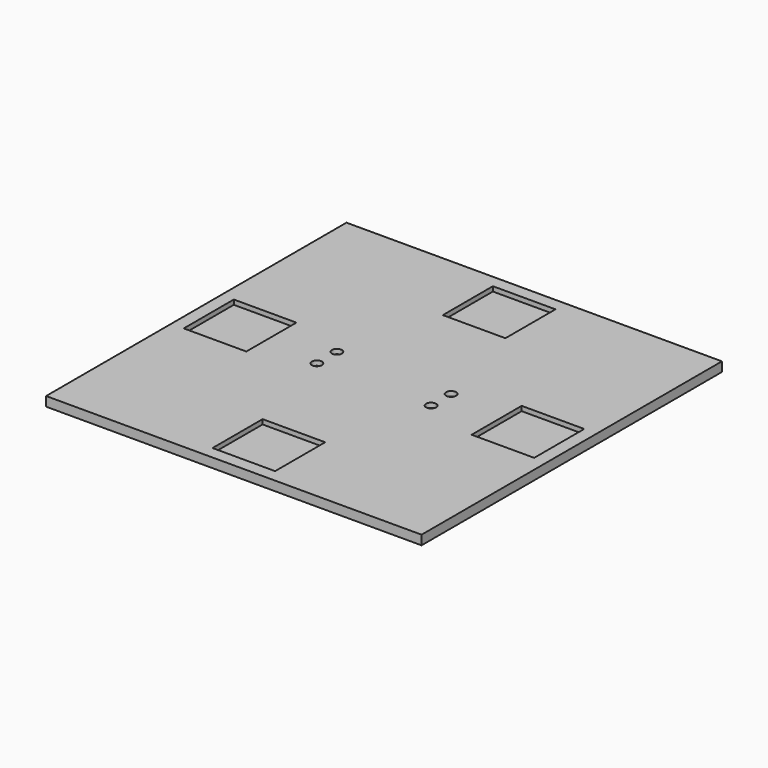
from build123d import *

# Parameters (mm, degrees)
F0_W             = 120
F0_H             = 120
F1_DEPTH         = 1.5
F5_W             = 120
F5_H             = 120
F5_W_2           = 112
F5_H_2           = 112
F6_DEPTH         = 1.5
F4_W             = 24
F4_H             = 24
F7_DEPTH         = 1.5
F7_COPIES_COUNT  = 4
F2_W             = 20
F2_H             = 20
F8_DEPTH         = 1.5
F8_COPIES_COUNT  = 4
F10_DEPTH        = 1.5
F12_DEPTH        = 1.5
F12_COPIES_COUNT = 4
F14_DEPTH        = 1.5
F14_COPIES_COUNT = 4
F16_R            = 1.6
F17_DEPTH        = 1.5


# Not quite as in the source:
# - a pattern or mirror of a feature is missing from the dataset's text; its kind, count and spacing are read off the source's solid


with BuildPart() as f1:
    # F0 (on Top) → F1 (new body)
    with BuildSketch(Plane.XY):
        Rectangle(F0_W, F0_H)
    extrude(amount=F1_DEPTH)

    # F5 (on face) → F6 (join)
    with BuildSketch(Plane(origin=(0, 0, 0), x_dir=(1, 0, 0), z_dir=(0, 0, -1))):
        Rectangle(F5_W, F5_H)
        Rectangle(F5_W_2, F5_H_2, mode=Mode.SUBTRACT)
    extrude(amount=F6_DEPTH)

    # F4 (on face) → F7 (join)
    with BuildSketch(Plane(origin=(0, 0, 0), x_dir=(1, 0, 0), z_dir=(0, 0, -1))):
        with Locations((0, -46)):
            Rectangle(F4_W, F4_H)
    f7 = extrude(amount=F7_DEPTH)

    # F7_copies: F7 ×4 about axis
    f7_copies_axis = Axis((0, 0, 0), (0, 0, 1))
    for i in range(1, F7_COPIES_COUNT):
        add(f7.rotate(f7_copies_axis, i * 360 / F7_COPIES_COUNT))

    # F2 (on face) → F8 (cut)
    with BuildSketch(Plane.XY.offset(1.5)):
        with Locations((0, 46)):
            Rectangle(F2_W, F2_H)
    f8 = extrude(amount=-F8_DEPTH, mode=Mode.SUBTRACT)

    # F8_copies: F8 ×4 about axis
    f8_copies_axis = Axis((0, 0, 0), (0, 0, 1))
    for i in range(1, F8_COPIES_COUNT):
        add(f8.rotate(f8_copies_axis, i * 360 / F8_COPIES_COUNT), mode=Mode.SUBTRACT)

    # F9 (on face) → F10 (join)
    with BuildSketch(Plane(origin=(0, 0, 0), x_dir=(1, 0, 0), z_dir=(0, 0, -1))):
        Polygon((-56, 56), (-56, 53.1715728753), (53.1715728753, -56), (56, -56), (56, -53.1715728753), (-53.1715728753, 56), align=None)
    f10 = extrude(amount=F10_DEPTH)

    # F10_copies: F10 across plane
    add(f10.mirror(Plane(origin=(0, 0, 0), x_dir=(0, 0, -1), z_dir=(-1, 0, 0))))

    # F11 (on face) → F12 (join)
    with BuildSketch(Plane(origin=(0, 0, 0), x_dir=(1, 0, 0), z_dir=(0, 0, -1))):
        Polygon((34, 9.1715728753), (34, 12), (36.8284271247, 12), (25.8284271247, 23), (23, 20.1715728753), align=None)
    f12 = extrude(amount=F12_DEPTH)

    # F12_copies: F12 ×4 about axis
    f12_copies_axis = Axis((0, 0, 0), (0, 0, 1))
    for i in range(1, F12_COPIES_COUNT):
        add(f12.rotate(f12_copies_axis, i * 360 / F12_COPIES_COUNT))

    # F13 (on face) → F14 (join)
    with BuildSketch(Plane(origin=(0, 0, 0), x_dir=(1, 0, 0), z_dir=(0, 0, -1))):
        Polygon((12, 36.8284271247), (12, 34), (9.1715728753, 34), (20.1715728753, 23), (23, 25.8284271247), align=None)
    f14 = extrude(amount=F14_DEPTH)

    # F14_copies: F14 ×4 about axis
    f14_copies_axis = Axis((0, 0, 0), (0, 0, 1))
    for i in range(1, F14_COPIES_COUNT):
        add(f14.rotate(f14_copies_axis, i * 360 / F14_COPIES_COUNT))

    # F16 (on face) → F17 (cut)
    with BuildSketch(Plane.XY.offset(1.5)):
        with Locations((18.25, 4)):
            Circle(F16_R)
        with Locations((18.25, -4)):
            Circle(F16_R)
        with Locations((-18.25, -4)):
            Circle(F16_R)
        with Locations((-18.25, 4)):
            Circle(F16_R)
    extrude(amount=-F17_DEPTH, mode=Mode.SUBTRACT)


solid = f1.part
